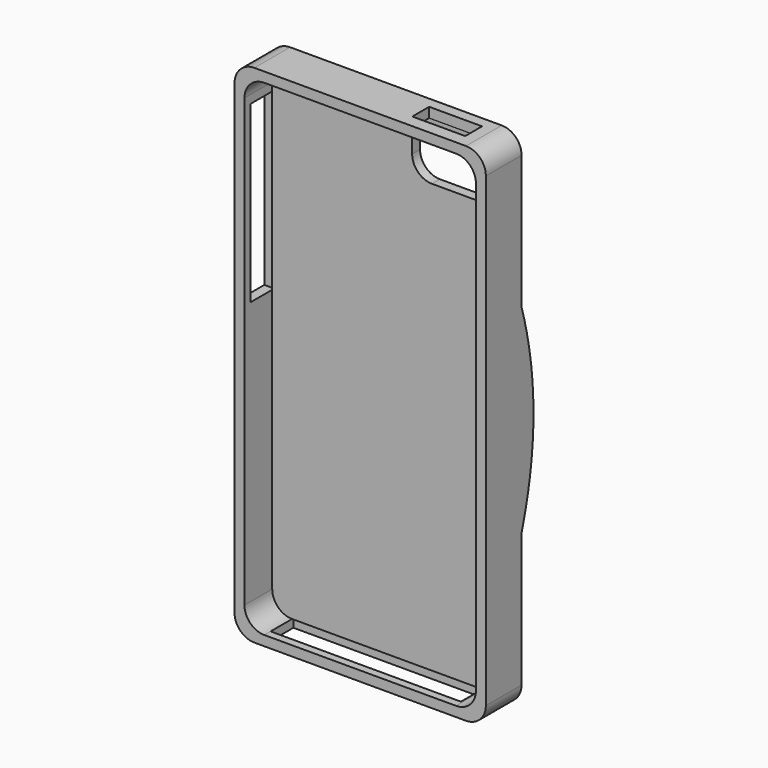
from build123d import *

# Parameters (mm, degrees)
F0_W          = 64.3382
F0_H          = 129.54
F1_DEPTH      = 11.43
F2_T          = -2.54
F3_R          = 5.08
F4_R          = 5.08
F5_W          = 49.1753579962
F5_H          = 7.874
F6_DEPTH      = 2.54
F7_W          = 7.62
F7_H          = 44.7040022942
F8_DEPTH      = 2.54
F9_W          = 13.5422451422
F9_H          = 5.387768615
F10_DEPTH     = 2.54
F11_W         = 20.9040842336
F11_H         = 12.1967079258
F12_DEPTH     = 2.54
F13_R         = 5.08
F16_W         = 15.2080394328
F16_H         = 50.8793298835
F17_DEPTH     = 13.97
F18_W         = 10.3803684741
F18_H         = 48.4102021849
F19_DEPTH     = 11.43
F22_DEPTH     = 25.4
F23_DEPTH     = 13.716
F25_DEPTH     = 25.4
F27_DEPTH     = 11.176
F28_TEXT_SIZE = 21.1877350146
F29_DEPTH     = 3.302
F30_TEXT_SIZE = 32.44525546
F31_DEPTH     = 11.684


# Not quite as in the source:
# - Text() gives the source's letters only with a copy of the font that has no kerning and outlines rounded to 1/6400 em; it was checked with that copy


with BuildPart() as f1:
    # F0 (on Front) → F1 (new body)
    with BuildSketch(Plane.XZ):
        with Locations((-0.4763082698, -0.0230428386)):
            Rectangle(F0_W, F0_H)
    extrude(amount=F1_DEPTH)

    # F2
    f2_openings = [f1.faces().sort_by_distance(p)[0] for p in [
        (-0.476308, -11.43, -0.023043),
    ]]
    offset(amount=F2_T, openings=f2_openings)

    # F3
    f3_edges = [f1.edges().sort_by_distance(p)[0] for p in [
        (-30.105408, -6.985, 62.206957),
        (29.152792, -6.985, 62.206957),
        (31.692792, -5.715, 64.746957),
        (-32.645408, -5.715, 64.746957),
    ]]
    fillet(f3_edges, radius=F3_R)

    # F4
    f4_edges = [f1.edges().sort_by_distance(p)[0] for p in [
        (-32.645408, -5.715, -64.793043),
        (31.692792, -5.715, -64.793043),
        (29.152792, -6.985, -62.253043),
        (-30.105408, -6.985, -62.253043),
    ]]
    fillet(f4_edges, radius=F4_R)

    # F5 (on face) → F6 (cut)
    with BuildSketch(Plane(origin=(0, 0, -64.7930428386), x_dir=(1, 0, 0), z_dir=(0, 0, -1))):
        with Locations((-0.8962145075, 5.4786364199)):
            Rectangle(F5_W, F5_H)
    extrude(amount=-F6_DEPTH, mode=Mode.SUBTRACT)

    # F7 (on face) → F8 (cut)
    with BuildSketch(Plane(origin=(-32.6454082698, 0, 0), x_dir=(0, -1, 0), z_dir=(-1, 0, 0))):
        with Locations((5.7087146561, 32.6503398828)):
            Rectangle(F7_W, F7_H)
    extrude(amount=-F8_DEPTH, mode=Mode.SUBTRACT)

    # F9 (on face) → F10 (cut)
    with BuildSketch(Plane.XY.offset(64.7469571614)):
        with Locations((17.0274716802, -5.4679538589)):
            Rectangle(F9_W, F9_H)
    extrude(amount=-F10_DEPTH, mode=Mode.SUBTRACT)

    # F11 (on face) → F12 (cut)
    with BuildSketch(Plane(origin=(0, 0, 0), x_dir=(-1, 0, 0), z_dir=(0, 1, 0))):
        with Locations((-16.1607496133, 53.5686031985)):
            Rectangle(F11_W, F11_H)
    extrude(amount=-F12_DEPTH, mode=Mode.SUBTRACT)

    # F13
    f13_edges = [f1.edges().sort_by_distance(p)[0] for p in [
        (26.612792, -1.27, 59.666957),
        (5.708707, -1.27, 47.470249),
    ]]
    fillet(f13_edges, radius=F13_R)

    # F14 (on Right) → F15 (revolve)
    with BuildSketch(Plane.YZ):
        with BuildLine():
            Line((0, 40.64), (0, 0))
            Line((0, 0), (10.6080601498, 0))
            ThreePointArc((10.6080601498, 0), (7.2584939174, 20.8301641241), (0, 40.64))
        make_face()
    revolve(axis=Axis((0, 5.3040300749, 0), (0, 1, 0)))

    # F16 (on face) → F17 (cut)
    with BuildSketch(Plane.XZ):
        with Locations((39.2968114465, 0)):
            Rectangle(F16_W, F16_H)
    extrude(amount=-F17_DEPTH, mode=Mode.SUBTRACT)

    # F18 (on face) → F19 (cut)
    with BuildSketch(Plane.XZ):
        with Locations((-37.8355925069, 0)):
            Rectangle(F18_W, F18_H)
    extrude(amount=-F19_DEPTH, mode=Mode.SUBTRACT)

    # F20 (on Front) → F22 (cut)
    with BuildSketch(Plane.XZ):
        with BuildLine():
            Line((-26.7186705023, -30.2227549255), (-24.3826080114, -31.682793051))
            ThreePointArc((-24.3826080114, -31.682793051), (-12.9760604048, 0.6298860355), (-23.7985923886, 33.1428274512))
            Line((-23.7985923886, 33.1428274512), (-25.8575548537, 31.3126436198))
            ThreePointArc((-25.8575548537, 31.3126436198), (-15.4242345843, 0.3929171295), (-26.7186705023, -30.2227549255))
        make_face()
    extrude(amount=-F22_DEPTH, mode=Mode.SUBTRACT)

    # F21 (on Front) → F23 (cut)
    with BuildSketch(Plane.XZ):
        with BuildLine():
            ThreePointArc((26.3857204148, -30.8386584448), (14.3504288371, -0.6047719665), (27.5497492403, 29.1393715888))
            Line((27.5497492403, 29.1393715888), (26.2218378484, 31.4694158733))
            ThreePointArc((26.2218378484, 31.4694158733), (12.228970635, -0.0096128734), (24.7761905193, -32.09226951))
            Line((24.7761905193, -32.09226951), (26.3857204148, -30.8386584448))
        make_face()
    extrude(amount=-F23_DEPTH, mode=Mode.SUBTRACT)

    # F24 (on Front) → F25 (cut)
    with BuildSketch(Plane.XZ):
        with BuildLine():
            ThreePointArc((18.5087900609, 12.5202322379), (15.5398408881, 12.7784859212), (13.3297918364, 14.7777451202))
            Line((13.3297918364, 14.7777451202), (12.7986129373, 13.8481808826))
            ThreePointArc((12.7986129373, 13.8481808826), (15.1780332757, 11.6083082636), (18.4423923492, 11.4578744397))
            Line((18.4423923492, 11.4578744397), (18.5087900609, 12.5202322379))
        make_face()
        with BuildLine():
            ThreePointArc((17.0303694904, 8.2456273958), (14.2928548871, 8.242580384), (12.0519287884, 9.8149180412))
            Line((12.0519287884, 9.8149180412), (11.510794051, 9.1655571014))
            ThreePointArc((11.510794051, 9.1655571014), (13.9120970482, 7.1701737333), (17.0303694904, 7.3256981559))
            Line((17.0303694904, 7.3256981559), (17.0303694904, 8.2456273958))
        make_face()
        with BuildLine():
            ThreePointArc((16.2182468921, 3.8993796334), (13.5384646856, 3.5792576819), (11.0971722752, 4.729823675))
            Line((11.0971722752, 4.729823675), (10.6127467006, 4.1761943139))
            ThreePointArc((10.6127467006, 4.1761943139), (13.3102736827, 2.7177250604), (16.3566544652, 3.0689351261))
            Line((16.3566544652, 3.0689351261), (16.2182468921, 3.8993796334))
        make_face()
        with BuildLine():
            ThreePointArc((16.1419343203, 0), (13.1847682636, -0.3944789715), (10.3809908032, 0.6249702419))
            Line((10.3809908032, 0.6249702419), (10.1594151929, -0.3942737821))
            ThreePointArc((10.1594151929, -0.3942737821), (13.0578171026, -1.3811748608), (16.0976182669, -1.0146830464))
            Line((16.0976182669, -1.0146830464), (16.1419343203, 0))
        make_face()
        with BuildLine():
            ThreePointArc((15.9748699516, -3.9926506579), (13.1913426711, -4.7960974735), (10.4843014851, -3.7638770882))
            Line((10.4843014851, -3.7638770882), (10.198334232, -4.6217786148))
            ThreePointArc((10.198334232, -4.6217786148), (13.1691063438, -5.5730861394), (16.2036437541, -4.8505519517))
            Line((16.2036437541, -4.8505519517), (15.9748699516, -3.9926506579))
        make_face()
        with BuildLine():
            ThreePointArc((16.5477115661, -7.4009019881), (13.7997036714, -8.4713974883), (10.9154647216, -7.8560328111))
            Line((10.9154647216, -7.8560328111), (10.6878988445, -8.6525129154))
            ThreePointArc((10.6878988445, -8.6525129154), (13.8760393495, -9.4569500623), (16.8890599161, -8.1404903904))
            Line((16.8890599161, -8.1404903904), (16.5477115661, -7.4009019881))
        make_face()
        with BuildLine():
            ThreePointArc((17.413392663, -11.1640626565), (14.5025263271, -12.3509346802), (11.4119304344, -11.7764566094))
            Line((11.4119304344, -11.7764566094), (11.1669730395, -12.3509346802))
            ThreePointArc((11.1669730395, -12.3509346802), (14.5797300113, -13.2356156997), (17.8420692682, -11.8989357725))
            Line((17.8420692682, -11.8989357725), (17.413392663, -11.1640626565))
        make_face()
        with BuildLine():
            ThreePointArc((22.8783134371, -23.7157624215), (20.4526797886, -25.7765041906), (17.2731429338, -25.9210746735))
            Line((17.2731429338, -25.9210746735), (17.5097901374, -27.2075068206))
            ThreePointArc((17.5097901374, -27.2075068206), (21.1659687288, -26.7848527864), (23.85058254, -24.2670904845))
            Line((23.85058254, -24.2670904845), (22.8783134371, -23.7157624215))
        make_face()
        with BuildLine():
            ThreePointArc((25.5047045648, -27.6669468731), (23.5382647588, -29.7218704208), (20.7261350006, -30.1479250193))
            Line((20.7261350006, -30.1479250193), (20.818028599, -31.1586931348))
            ThreePointArc((20.818028599, -31.1586931348), (23.9903132267, -30.6858698946), (26.3317637146, -28.4939389676))
            Line((26.3317637146, -28.4939389676), (25.5047045648, -27.6669468731))
        make_face()
        with BuildLine():
            ThreePointArc((18.39488931, -15.91909118), (16.0583442356, -17.4041016712), (13.2933044806, -17.265342176))
            Line((13.2933044806, -17.265342176), (13.1515935063, -18.1864630431))
            ThreePointArc((13.1515935063, -18.1864630431), (16.266591513, -18.3386141577), (18.9617332071, -16.769355163))
            Line((18.9617332071, -16.769355163), (18.39488931, -15.91909118))
        make_face()
        with BuildLine():
            ThreePointArc((20.0245641172, -19.6035690606), (17.6740869872, -21.2919294989), (14.7812664509, -21.3749539107))
            Line((14.7812664509, -21.3749539107), (15.1355434209, -22.5086398423))
            ThreePointArc((15.1355434209, -22.5086398423), (18.1772730598, -22.2921263141), (20.6622611731, -20.5246899277))
            Line((20.6622611731, -20.5246899277), (20.0245641172, -19.6035690606))
        make_face()
        with BuildLine():
            Line((15.4409334064, 19.0867930651), (14.709006995, 18.2633753866))
            ThreePointArc((14.709006995, 18.2633753866), (16.4239444356, 16.1216646792), (19.1005673259, 15.5186513439))
            Line((19.1005673259, 15.5186513439), (19.2835479975, 16.6165418923))
            ThreePointArc((19.2835479975, 16.6165418923), (16.9242153716, 17.170294449), (15.4409334064, 19.0867930651))
        make_face()
        with BuildLine():
            Line((17.3622407019, 22.5634444505), (16.4239444356, 22.1059899777))
            ThreePointArc((16.4239444356, 22.1059899777), (18.4427089979, 19.8959531308), (21.3878378272, 19.3612668663))
            Line((21.3878378272, 19.3612668663), (21.4793272316, 20.3676652163))
            ThreePointArc((21.4793272316, 20.3676652163), (19.0265676837, 20.7263992191), (17.3622407019, 22.5634444505))
        make_face()
        with BuildLine():
            Line((20.0154744089, 25.7656238973), (19.1005673259, 25.3996606916))
            ThreePointArc((19.1005673259, 25.3996606916), (20.6346852724, 23.1354944346), (23.3091432601, 22.5634444505))
            Line((23.3091432601, 22.5634444505), (23.858089, 23.4783533961))
            ThreePointArc((23.858089, 23.4783533961), (21.5681967245, 24.0027658564), (20.0154744089, 25.7656238973))
        make_face()
        with BuildLine():
            Line((22.6687081158, 28.8763102144), (21.7538010329, 28.6018382758))
            ThreePointArc((21.7538010329, 28.6018382758), (22.9430482325, 26.435405106), (25.3219418228, 25.7656238973))
            Line((25.3219418228, 25.7656238973), (26.0538682342, 26.5890397131))
            ThreePointArc((26.0538682342, 26.5890397131), (23.9374770393, 27.1054345243), (22.6687081158, 28.8763102144))
        make_face()
    extrude(amount=-F25_DEPTH, mode=Mode.SUBTRACT)

    # F26 (on Front) → F27 (cut)
    with BuildSketch(Plane.XZ):
        with BuildLine():
            ThreePointArc((-19.2867424339, 30.8206696063), (-22.009359823, 28.918710309), (-25.1825097948, 27.9382951558))
            Line((-25.1825097948, 27.9382951558), (-25.1825097948, 26.6268625855))
            ThreePointArc((-25.1825097948, 26.6268625855), (-21.5590275704, 27.6010014338), (-18.4998456389, 29.7735519707))
            Line((-18.4998456389, 29.7735519707), (-19.2867424339, 30.8206696063))
        make_face()
        with BuildLine():
            ThreePointArc((-17.2312991077, 26.2879002902), (-19.6744197454, 24.4877896873), (-22.6351190358, 23.8218344748))
            Line((-22.6351190358, 23.8218344748), (-22.3370008171, 22.8284485638))
            ThreePointArc((-22.3370008171, 22.8284485638), (-19.2917664267, 23.6123763632), (-16.6350626701, 25.2946130994))
            Line((-16.6350626701, 25.2946130994), (-17.2312991077, 26.2879002902))
        make_face()
        with BuildLine():
            ThreePointArc((-14.9779301137, 21.8998026103), (-17.448145216, 20.2597923187), (-20.4124432057, 20.1924585479))
            Line((-20.4124432057, 20.1924585479), (-20.4124432057, 18.7286660075))
            ThreePointArc((-20.4124432057, 18.7286660075), (-17.1389390368, 19.0433919817), (-14.411835, 20.8812672645))
            Line((-14.411835, 20.8812672645), (-14.9779301137, 21.8998026103))
        make_face()
        with BuildLine():
            ThreePointArc((-11.3222306609, 5.7809644024), (-14.2195968718, 4.7708817044), (-17.2595394483, 5.1877115845))
            Line((-17.2595394483, 5.1877115845), (-17.9383591273, 4.1210347615))
            ThreePointArc((-17.9383591273, 4.1210347615), (-14.2804197992, 3.6766850253), (-10.821243991, 4.9463580318))
            Line((-10.821243991, 4.9463580318), (-11.3222306609, 5.7809644024))
        make_face()
        with BuildLine():
            ThreePointArc((-14.1109625223, -17.4193982867), (-17.5449948419, -16.989106649), (-20.4251003821, -15.070064976))
            Line((-20.4251003821, -15.070064976), (-21.3975909791, -16.1641173697))
            ThreePointArc((-21.3975909791, -16.1641173697), (-18.1425098719, -18.3991448212), (-14.2232298852, -18.8788792357))
            Line((-14.2232298852, -18.8788792357), (-14.1109625223, -17.4193982867))
        make_face()
        with BuildLine():
            ThreePointArc((-20.4664105928, -30.1615360597), (-24.1507789625, -28.7313607922), (-26.6282465309, -25.6520546973))
            Line((-26.6282465309, -25.6520546973), (-27.8274640441, -26.49143897))
            ThreePointArc((-27.8274640441, -26.49143897), (-25.0557707219, -29.8864869039), (-20.9919176996, -31.5277464688))
            Line((-20.9919176996, -31.5277464688), (-20.4664105928, -30.1615360597))
        make_face()
        with BuildLine():
            ThreePointArc((-17.5162758678, -24.7129869396), (-20.9297579941, -23.8214620577), (-23.3829381307, -21.2859968028))
            Line((-23.3829381307, -21.2859968028), (-24.4180385506, -22.3210116441))
            ThreePointArc((-24.4180385506, -22.3210116441), (-21.5348007699, -25.2649684459), (-17.5162758678, -26.1767794799))
            Line((-17.5162758678, -26.1767794799), (-17.5162758678, -24.7129869396))
        make_face()
        with BuildLine():
            ThreePointArc((-13.6131718755, 16.387994329), (-16.2209015037, 15.0394359905), (-19.1403906792, 15.348379934))
            Line((-19.1403906792, 15.348379934), (-19.1403906792, 13.8845873937))
            ThreePointArc((-19.1403906792, 13.8845873937), (-15.6624079783, 13.5807552682), (-12.7891948889, 15.5640162626))
            Line((-12.7891948889, 15.5640162626), (-13.6131718755, 16.387994329))
        make_face()
        with BuildLine():
            ThreePointArc((-11.2377908081, 0), (-14.139238745, -0.4194765781), (-17.0406866819, 0))
            Line((-17.0406866819, 0), (-17.363069579, -0.7236557431))
            ThreePointArc((-17.363069579, -0.7236557431), (-14.1852935776, -1.2728403284), (-11.0075175762, -0.7236557431))
            Line((-11.0075175762, -0.7236557431), (-11.2377908081, 0))
        make_face()
        with BuildLine():
            ThreePointArc((-11.9543063205, 11.2185046657), (-14.6928273654, 10.1829145185), (-17.6178905787, 10.3092065019))
            Line((-17.6178905787, 10.3092065019), (-18.1000850087, 9.2483735933))
            ThreePointArc((-18.1000850087, 9.2483735933), (-14.6242372747, 8.952205061), (-11.3704576762, 10.2100411368))
            Line((-11.3704576762, 10.2100411368), (-11.9543063205, 11.2185046657))
        make_face()
        with BuildLine():
            ThreePointArc((-11.5476373644, -5.3490266507), (-14.8082087085, -6.1098228311), (-18.0038042261, -5.110670387))
            Line((-18.0038042261, -5.110670387), (-18.5874139273, -5.9860854211))
            ThreePointArc((-18.5874139273, -5.9860854211), (-15.0021245491, -7.0593012075), (-11.2938579923, -6.5544733225))
            Line((-11.2938579923, -6.5544733225), (-11.5476373644, -5.3490266507))
        make_face()
        with BuildLine():
            ThreePointArc((-12.8402798651, -11.4423090942), (-15.9218740344, -11.5099730264), (-18.6546072364, -10.084150359))
            Line((-18.6546072364, -10.084150359), (-19.4496810436, -10.7732145116))
            ThreePointArc((-19.4496810436, -10.7732145116), (-16.2726440444, -12.5959775437), (-12.6120429486, -12.4693727121))
            Line((-12.6120429486, -12.4693727121), (-12.8402798651, -11.4423090942))
        make_face()
    extrude(amount=-F27_DEPTH, mode=Mode.SUBTRACT)

    # F28 (on face) → F29 (join)
    with BuildSketch(Plane(origin=(0, 0, 0), x_dir=(-1, 0, 0), z_dir=(0, 1, 0))):
        with Locations((-30.2854753072, -59.7130428386)):
            Text('Foster', F28_TEXT_SIZE, font='Open Sans', text_align=(TextAlign.LEFT, TextAlign.BOTTOM))
    extrude(amount=F29_DEPTH)

    # F30 (on face) → F31 (join)
    with BuildSketch(Plane(origin=(0, 0, 0), x_dir=(-1, 0, 0), z_dir=(0, 1, 0))):
        with Locations((-8.9062238112, -12.3509346802)):
            Text('6', F30_TEXT_SIZE, font='Open Sans', font_style=FontStyle.BOLD, text_align=(TextAlign.LEFT, TextAlign.BOTTOM))
    extrude(amount=F31_DEPTH)


solid = f1.part
